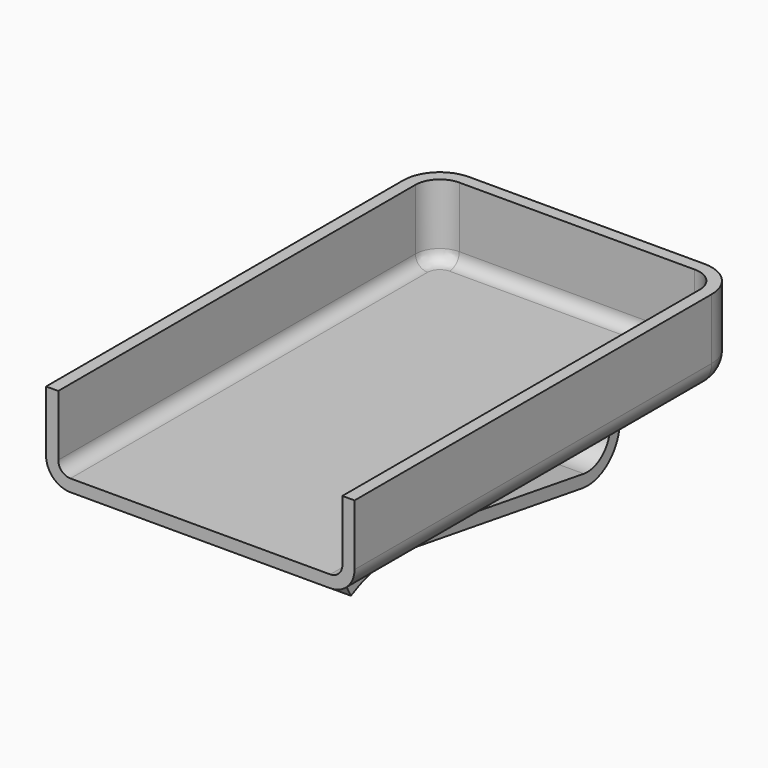
from build123d import *

# Parameters (mm, degrees)
F0_W        = 38
F0_H        = 59.5
F1_DEPTH    = 10.5
F2_R        = 3
F3_T1_DEPTH = 21.75
F3_T4_ANGLE = 90
F3_T6_ANGLE = 90
F4_T        = -1.5
F6_DEPTH    = 10


# Not quite as in the source:
# - a fillet or chamfer that OpenCascade refuses, or shapes differently, is made with other operations: its cross-section is extruded or revolved along the edge and cut away or added


with BuildPart() as f1:
    # F0 (on Top) → F1 (new body)
    with BuildSketch(Plane.XY):
        with Locations((0, 29.75)):
            Rectangle(F0_W, F0_H)
    extrude(amount=F1_DEPTH)

    # F2
    f2_edges = [f1.edges().sort_by_distance(p)[0] for p in [
        (19, 29.75, 0),
        (0, 59.5, 0),
        (-19, 29.75, 0),
    ]]
    fillet(f2_edges, radius=F2_R)

    # F3: fillet of radius 4.5 on 2 edges, made by hand

    # F3_s2 → F3_t1 (cut)
    with BuildSketch(Plane.XY):
        with BuildLine():
            ThreePointArc((14.5, 59.5), (17.6819805153, 58.1819805153), (19, 55))
            Line((19, 55), (19, 59.5))
            Line((19, 59.5), (14.5, 59.5))
        make_face()
        with BuildLine():
            ThreePointArc((-19, 55), (-17.6819805153, 58.1819805153), (-14.5, 59.5))
            Line((-14.5, 59.5), (-19, 59.5))
            Line((-19, 59.5), (-19, 55))
        make_face()
    extrude(amount=F3_T1_DEPTH, mode=Mode.SUBTRACT)

    # F3_s3 → F3_t4 (revolve, cut)
    with BuildSketch(Plane.XZ.offset(-55)):
        with BuildLine():
            ThreePointArc((-16, 0), (-18.1213203436, 0.8786796564), (-19, 3))
            Line((-19, 3), (-19, 0))
            Line((-19, 0), (-16, 0))
        make_face()
    revolve(axis=Axis((-14.5, 55, 0), (0, 0, -1)), revolution_arc=F3_T4_ANGLE, mode=Mode.SUBTRACT)

    # F3_s5 → F3_t6 (revolve, cut)
    with BuildSketch(Plane.YZ.offset(14.5)):
        with BuildLine():
            ThreePointArc((56.5, 0), (58.6213203436, 0.8786796564), (59.5, 3))
            Line((59.5, 3), (59.5, 0))
            Line((59.5, 0), (56.5, 0))
        make_face()
    revolve(axis=Axis((14.5, 55, 0), (0, 0, -1)), revolution_arc=F3_T6_ANGLE, mode=Mode.SUBTRACT)

    # F4
    f4_openings = [f1.faces().sort_by_distance(p)[0] for p in [
        (0, 0, 5.294773),
        (0, 29.639077, 10.5),
    ]]
    offset(amount=F4_T, openings=f4_openings)

    # F5 (on Right) → F6 (join, symmetric)
    with BuildSketch(Plane.YZ):
        with BuildLine():
            ThreePointArc((46.3163853092, -9.9390293558), (52.0795723104, -5.3904185068), (47.0948382764, 0))
            Line((47.0948382764, 0), (9.9783393557, 0))
            Line((9.9783393557, 0), (9.9783393557, -1.5))
            Line((9.9783393557, -1.5), (47.0948382764, -1.5))
            ThreePointArc((47.0948382764, -1.5), (50.5841521002, -5.2732929547), (46.5499211994, -8.4573205491))
            Line((46.5499211994, -8.4573205491), (19.4301971783, -4.1829119325))
            ThreePointArc((19.4301971783, -4.1829119325), (14.5719355532, -4.213690053), (9.9783393557, -5.795627879))
            Line((9.9783393557, -5.795627879), (10.6899892478, -7.1160650911))
            ThreePointArc((10.6899892478, -7.1160650911), (14.8242258255, -5.6923210477), (19.1966612881, -5.6646207393))
            Line((19.1966612881, -5.6646207393), (46.3163853092, -9.9390293558))
        make_face()
    extrude(amount=F6_DEPTH, both=True)


solid = f1.part
